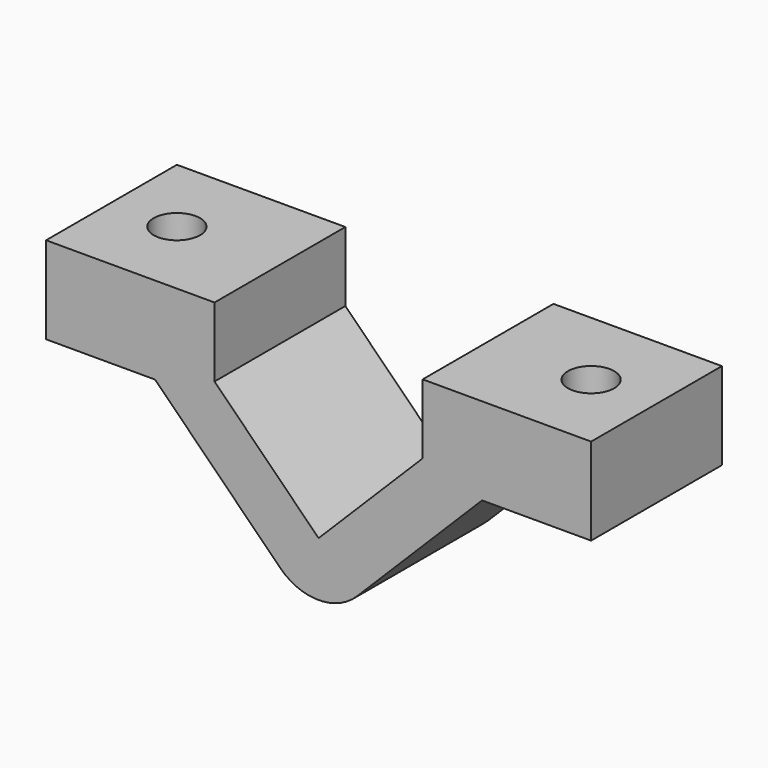
from build123d import *

# Parameters (mm, degrees)
F1_DEPTH = 15
F2_R     = 2.125
F3_DEPTH = 25
F5_DEPTH = 4
F6_R     = 5
F8_DEPTH = 25


# Not quite as in the source:
# - a feature names something its author has since deleted; it is built from what else it names


with BuildPart() as f1:
    # F0 (on Front) → F1 (new body)
    with BuildSketch(Plane.XZ):
        Polygon((25, 12.8176623509), (15, 12.8176623509), (9.545941546, 12.8176623509), (9.545941546, 6.4346717088), (0, -3.1112698372), (-9.545941546, 6.4346717088), (-9.545941546, 12.8176623509), (-15, 12.8176623509), (-25, 12.8176623509), (-25, 4.8176623509), (-15, 4.8176623509), (-7.5, -2.6823376491), (0, -10.1823376491), (7.5, -2.6823376491), (15, 4.8176623509), (25, 4.8176623509), align=None)
    extrude(amount=F1_DEPTH)

    # F2 (on face) → F3 (cut)
    with BuildSketch(Plane.XY.offset(12.8176623509)):
        with Locations((-19, -7.5)):
            Circle(F2_R)
        with Locations((19, -7.5)):
            Circle(F2_R)
    extrude(amount=-F3_DEPTH, mode=Mode.SUBTRACT)

    # F4 (on face) → F5 (cut)
    with BuildSketch(Plane(origin=(0, 0, 4.8176623509), x_dir=(1, 0, 0), z_dir=(0, 0, -1))):
        Polygon((-21.925, 9.1887495374), (-21.925, 5.8112504626), (-19, 4.1225009252), (-16.075, 5.8112504626), (-16.075, 9.1887495374), (-19, 10.8774990748), align=None)
        Polygon((21.925, 5.8112504626), (21.925, 9.1887495374), (19, 10.8774990748), (16.075, 9.1887495374), (16.075, 5.8112504626), (19, 4.1225009252), align=None)
    extrude(amount=-F5_DEPTH, mode=Mode.SUBTRACT)

    # F6
    f6_edges = [f1.edges().sort_by_distance(p)[0] for p in [
        (0, -7.5, -10.182338),
    ]]
    fillet(f6_edges, radius=F6_R)

    # F7 (on face) → F8 (cut)
    with BuildSketch(Plane(origin=(0, 0, 8.8176623509), x_dir=(1, 0, 0), z_dir=(0, 0, -1))):
        Polygon((-21.925, 9.1887495374), (-21.925, 5.8112504626), (-19, 4.1225009252), (-16.075, 5.8112504626), (-16.075, 9.1887495374), (-19, 10.8774990748), align=None)
    extrude(amount=F8_DEPTH, mode=Mode.SUBTRACT)


solid = f1.part
